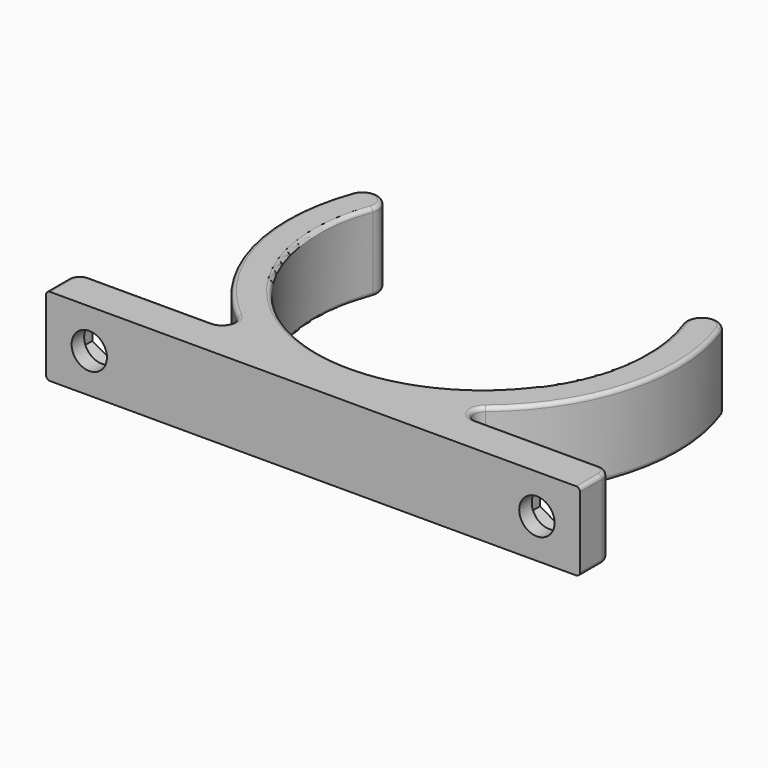
from build123d import *

# Parameters (mm, degrees)
F1_DEPTH  = 5
F2_R      = 2.25
F3_DEPTH  = 25
F5_DEPTH  = 3
F6_R      = 0.5
F7_R      = 0.5
F8_R      = 2.25
F9_DEPTH  = 25
F11_DEPTH = 3


# Not quite as in the source:
# - a feature names something its author has since deleted; it is built from what else it names


with BuildPart() as f1:
    # F0 (on Top) → F1 (new body, symmetric)
    with BuildSketch(Plane.XY):
        with BuildLine():
            Line((23.4923155196, 8.5505035831), (19.7335450365, 7.1824230098))
            ThreePointArc((19.7335450365, 7.1824230098), (0, -21), (-19.7335450365, 7.1824230098))
            Line((-19.7335450365, 7.1824230098), (-23.4923155196, 8.5505035831))
            ThreePointArc((-23.4923155196, 8.5505035831), (-24.1094573309, -6.6131737621), (-15.8420529306, -19.3398386483))
            ThreePointArc((-15.8420529306, -19.3398386483), (-15.380031471, -21.0049245713), (-16.792597972, -22.0002289671))
            Line((-16.792597972, -22.0002289671), (-32.5, -22))
            ThreePointArc((-32.5, -22), (-33.5606601718, -22.4393398282), (-34, -23.5))
            Line((-34, -23.5), (-34, -27))
            Line((-34, -27), (34, -27))
            Line((34, -27), (34, -23.5))
            ThreePointArc((34, -23.5), (33.5606601718, -22.4393398282), (32.5, -22))
            Line((32.5, -22), (16.7928556237, -22))
            ThreePointArc((16.7928556237, -22), (15.3803107505, -21.0046949387), (15.8423166262, -19.3396226415))
            ThreePointArc((15.8423166262, -19.3396226415), (24.1095024154, -6.6130093967), (23.4923155196, 8.5505035831))
        make_face()
        with BuildLine():
            Line((-23.4923155196, 8.5505035831), (-19.7335450365, 7.1824230098))
            ThreePointArc((-19.7335450365, 7.1824230098), (-20.9288899914, 9.7458485381), (-23.4923155196, 8.5505035831))
        make_face()
        with BuildLine():
            ThreePointArc((23.4923155196, 8.5505035831), (20.9288899914, 9.7458485381), (19.7335450365, 7.1824230098))
            Line((19.7335450365, 7.1824230098), (23.4923155196, 8.5505035831))
        make_face()
    extrude(amount=F1_DEPTH, both=True)

    # F2 (on face) → F3 (cut)
    with BuildSketch(Plane(origin=(0, -22, 0), x_dir=(-1, 0, 0), z_dir=(0, 1, 0))):
        with Locations((-28.5, 0)):
            Circle(F2_R)
    extrude(amount=-F3_DEPTH, mode=Mode.SUBTRACT)

    # F4 (on face) → F5 (cut)
    with BuildSketch(Plane(origin=(0, -22, 0), x_dir=(-1, 0, 0), z_dir=(0, 1, 0))):
        Polygon((-32.1, 2.0784609691), (-32.1, -2.0784609691), (-28.5, -4.1569219382), (-24.9, -2.0784609691), (-24.9, 2.0784609691), (-28.5, 4.1569219382), align=None)
    extrude(amount=-F5_DEPTH, mode=Mode.SUBTRACT)

    # F6
    f6_edges = [f1.edges().sort_by_distance(p)[0] for p in [
        (0, -21, 5),
        (20.92889, 9.745849, 5),
        (24.646428, -22, 5),
        (33.56066, -22.43934, 5),
        (34, -25.25, 5),
        (-20.92889, 9.745849, 5),
        (-33.56066, -22.43934, 5),
        (-34, -25.25, 5),
    ]]
    fillet(f6_edges, radius=F6_R)

    # F7
    f7_edges = [f1.edges().sort_by_distance(p)[0] for p in [
        (0, -21, -5),
        (20.92889, 9.745849, -5),
        (24.646428, -22, -5),
        (33.56066, -22.43934, -5),
        (34, -25.25, -5),
        (-20.92889, 9.745849, -5),
        (-33.56066, -22.43934, -5),
        (-34, -25.25, -5),
    ]]
    fillet(f7_edges, radius=F7_R)

    # F8 (on face) → F9 (cut)
    with BuildSketch(Plane(origin=(-0.0003207013, -22.0004737484, 0), x_dir=(-0.9999999999, 1.4577e-05, 0), z_dir=(1.4577e-05, 0.9999999999, 0))):
        with Locations((28.5, 0)):
            Circle(F8_R)
    extrude(amount=-F9_DEPTH, mode=Mode.SUBTRACT)

    # F10 (on face) → F11 (cut)
    with BuildSketch(Plane(origin=(-0.0003207013, -22.0004737484, 0), x_dir=(-0.9999999999, 1.4577e-05, 0), z_dir=(1.4577e-05, 0.9999999999, 0))):
        Polygon((32.1, -2.0784609691), (32.1, 2.0784609691), (28.5, 4.1569219382), (24.9, 2.0784609691), (24.9, -2.0784609691), (28.5, -4.1569219382), align=None)
    extrude(amount=-F11_DEPTH, mode=Mode.SUBTRACT)


solid = f1.part
